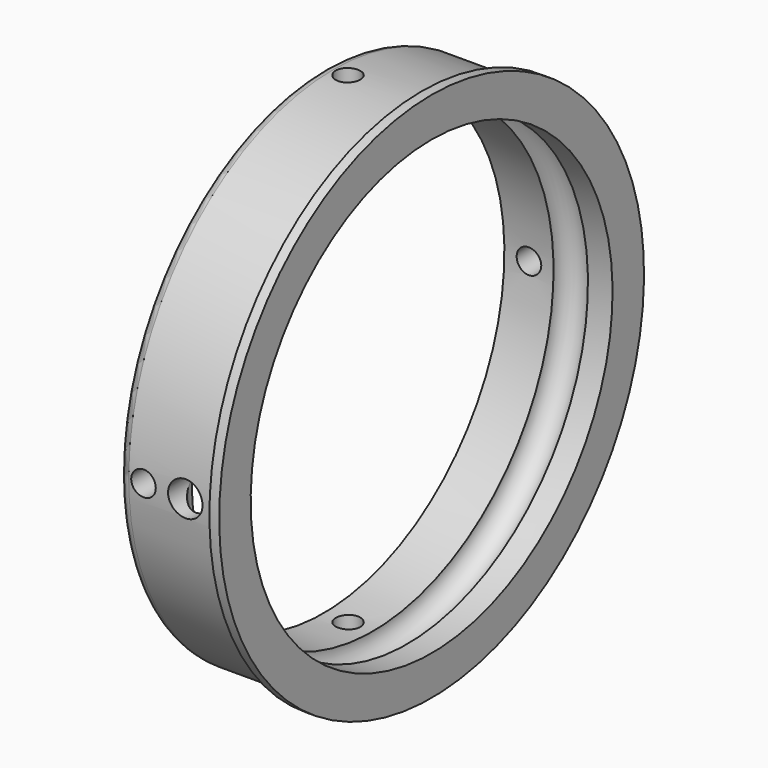
from build123d import *

# Parameters (mm, degrees)
F2_R          = 2
F3_R          = 3.5
F4_DEPTH      = 68.6
F5_R          = 2.5
F6_DEPTH      = 70.9
F6_DEPTH_BACK = 64.5
F7_R          = 2.5
F8_DEPTH      = 58.7
F8_DEPTH_BACK = 65.9


# Not quite as in the source:
# - a feature names something its author has since deleted; it is built from what else it names


with BuildPart() as f1:
    # F0 (on Front) → F1 (revolve)
    with BuildSketch(Plane.XZ):
        with BuildLine():
            Line((0, 46), (0, 54))
            Line((0, 54), (-2, 54))
            Line((-2, 54), (-2, 52))
            Line((-2, 52), (-22, 52))
            Line((-22, 52), (-22, 46))
            Line((-22, 46), (-12, 46))
            ThreePointArc((-12, 46), (-8.5, 49.5), (-5, 46))
            Line((-5, 46), (0, 46))
        make_face()
    revolve(axis=Axis((-49.1739120584, 0, 0), (-1, 0, 0)))

    # F2
    f2_edges = [f1.edges().sort_by_distance(p)[0] for p in [
        (-22, 0, -52),
    ]]
    fillet(f2_edges, radius=F2_R)

    # F3 (on Front) → F4 (cut)
    with BuildSketch(Plane.XZ):
        with Locations((-8.5, 0)):
            Circle(F3_R)
    extrude(amount=F4_DEPTH, mode=Mode.SUBTRACT)

    # F5 (on Top) → F6 (cut, two sides)
    with BuildSketch(Plane.XY) as f6_sk:
        with Locations((-17, 0)):
            Circle(F5_R)
    extrude(amount=F6_DEPTH, mode=Mode.SUBTRACT)
    extrude(f6_sk.sketch, amount=-F6_DEPTH_BACK, mode=Mode.SUBTRACT)

    # F7 (on Front) → F8 (cut, two sides)
    with BuildSketch(Plane.XZ) as f8_sk:
        with Locations((-17, 0)):
            Circle(F7_R)
    extrude(amount=F8_DEPTH, mode=Mode.SUBTRACT)
    extrude(f8_sk.sketch, amount=-F8_DEPTH_BACK, mode=Mode.SUBTRACT)


solid = f1.part
